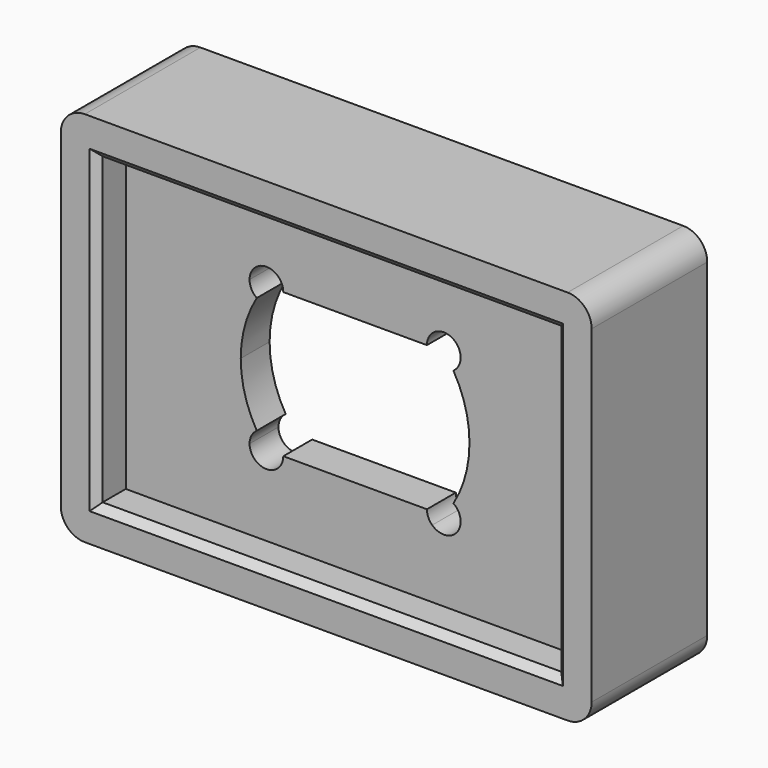
from build123d import *

# Parameters (mm, degrees)
F0_W     = 38.1
F0_H     = 25.3
F1_DEPTH = 3
F0_W_2   = 44.1
F0_H_2   = 31.3
F2_DEPTH = 6
F3_DEPTH = 6
F4_SIZE  = 0.6
F5_R     = 2


# Not quite as in the source:
# - a feature names something its author has since deleted; it is built from what else it names


with BuildPart() as f1:
    # F0 (on Front) → F1 (new body)
    with BuildSketch(Plane.XZ):
        Rectangle(F0_W, F0_H)
        with BuildLine():
            ThreePointArc((-8.6746757864, 9), (0, 12.5), (8.6746757864, 9))
            Line((8.6746757864, 9), (12.5, 9))
            Line((12.5, 9), (12.5, 0))
            Line((12.5, 0), (12.5, -9))
            Line((12.5, -9), (8.6746757864, -9))
            ThreePointArc((8.6746757864, -9), (0, -12.5), (-8.6746757864, -9))
            Line((-8.6746757864, -9), (-12.5, -9))
            Line((-12.5, -9), (-12.5, 0))
            Line((-12.5, 0), (-12.5, 9))
            Line((-12.5, 9), (-8.6746757864, 9))
        make_face(mode=Mode.SUBTRACT)
        with BuildLine():
            ThreePointArc((-3.0413812651, 9), (0, 9.5), (3.0413812651, 9))
            Line((3.0413812651, 9), (8.6746757864, 9))
            ThreePointArc((8.6746757864, 9), (0, 12.5), (-8.6746757864, 9))
            Line((-8.6746757864, 9), (-3.0413812651, 9))
        make_face()
        with BuildLine():
            ThreePointArc((12.5, 0), (11.5039872942, -4.8896090165), (8.6746757864, -9))
            Line((8.6746757864, -9), (12.5, -9))
            Line((12.5, -9), (12.5, 0))
        make_face()
        with BuildLine():
            Line((8.6746757864, -9), (3.0413812651, -9))
            ThreePointArc((3.0413812651, -9), (0, -9.5), (-3.0413812651, -9))
            Line((-3.0413812651, -9), (-8.6746757864, -9))
            ThreePointArc((-8.6746757864, -9), (0, -12.5), (8.6746757864, -9))
        make_face()
        with BuildLine():
            Line((-12.5, -9), (-8.6746757864, -9))
            ThreePointArc((-8.6746757864, -9), (-11.5039872942, -4.8896090165), (-12.5, 0))
            Line((-12.5, 0), (-12.5, -9))
        make_face()
        with BuildLine():
            Line((-3.0413812651, 9), (3.0413812651, 9))
            ThreePointArc((3.0413812651, 9), (0, 9.5), (-3.0413812651, 9))
        make_face()
        with BuildLine():
            ThreePointArc((-3.0413812651, -9), (0, -9.5), (3.0413812651, -9))
            Line((3.0413812651, -9), (-3.0413812651, -9))
        make_face()
        with BuildLine():
            ThreePointArc((-6.4036735124, 7.0173332219), (-4.8254540539, 8.1832141102), (-3.0413812651, 9))
            Line((-3.0413812651, 9), (-8.6746757864, 9))
            ThreePointArc((-8.6746757864, 9), (-11.5039872942, 4.8896090165), (-12.5, 0))
            ThreePointArc((-12.5, 0), (-11.5039872942, -4.8896090165), (-8.6746757864, -9))
            Line((-8.6746757864, -9), (-3.0413812651, -9))
            ThreePointArc((-3.0413812651, -9), (-4.8254540539, -8.1832141102), (-6.4036735124, -7.0173332219))
            ThreePointArc((-6.4036735124, -7.0173332219), (-7.9193096463, -7.2857878881), (-8.7654599313, -6))
            Line((-8.7654599313, -6), (-9.5, -6))
            Line((-9.5, -6), (-9.5, 0))
            Line((-9.5, 0), (-9.5, 6))
            Line((-9.5, 6), (-8.7654599313, 6))
            ThreePointArc((-8.7654599313, 6), (-7.9193096463, 7.2857878881), (-6.4036735124, 7.0173332219))
        make_face()
        with BuildLine():
            Line((9.5, 6), (9.5, 0))
            Line((9.5, 0), (9.5, -6))
            Line((9.5, -6), (8.7654599313, -6))
            ThreePointArc((8.7654599313, -6), (7.9193096463, -7.2857878881), (6.4036735124, -7.0173332219))
            ThreePointArc((6.4036735124, -7.0173332219), (4.8254540539, -8.1832141102), (3.0413812651, -9))
            Line((3.0413812651, -9), (8.6746757864, -9))
            ThreePointArc((8.6746757864, -9), (11.5039872942, -4.8896090165), (12.5, 0))
            ThreePointArc((12.5, 0), (11.5039872942, 4.8896090165), (8.6746757864, 9))
            Line((8.6746757864, 9), (3.0413812651, 9))
            ThreePointArc((3.0413812651, 9), (4.8254540539, 8.1832141102), (6.4036735124, 7.0173332219))
            ThreePointArc((6.4036735124, 7.0173332219), (7.9193096463, 7.2857878881), (8.7654599313, 6))
            Line((8.7654599313, 6), (9.5, 6))
        make_face()
        with BuildLine():
            Line((9.5, -6), (9.5, 0))
            ThreePointArc((9.5, 0), (9.1607649693, -2.5160256709), (8.1672873313, -4.852362069))
            ThreePointArc((8.1672873313, -4.852362069), (8.6069425852, -5.3529135915), (8.7654599313, -6))
            Line((8.7654599313, -6), (9.5, -6))
        make_face()
        with BuildLine():
            ThreePointArc((-8.7654599313, -6), (-8.6069425852, -5.3529135915), (-8.1672873313, -4.852362069))
            ThreePointArc((-8.1672873313, -4.852362069), (-9.1607649693, -2.5160256709), (-9.5, 0))
            Line((-9.5, 0), (-9.5, -6))
            Line((-9.5, -6), (-8.7654599313, -6))
        make_face()
        with BuildLine():
            ThreePointArc((-9.5, 0), (-9.1607649693, 2.5160256709), (-8.1672873313, 4.852362069))
            ThreePointArc((-8.1672873313, 4.852362069), (-8.6069425852, 5.3529135915), (-8.7654599313, 6))
            Line((-8.7654599313, 6), (-9.5, 6))
            Line((-9.5, 6), (-9.5, 0))
        make_face()
        with BuildLine():
            ThreePointArc((8.1672873313, 4.852362069), (9.1607649693, 2.5160256709), (9.5, 0))
            Line((9.5, 0), (9.5, 6))
            Line((9.5, 6), (8.7654599313, 6))
            ThreePointArc((8.7654599313, 6), (8.6069425852, 5.3529135915), (8.1672873313, 4.852362069))
        make_face()
        with BuildLine():
            ThreePointArc((-12.5, 0), (-11.5039872942, 4.8896090165), (-8.6746757864, 9))
            Line((-8.6746757864, 9), (-12.5, 9))
            Line((-12.5, 9), (-12.5, 0))
        make_face()
        with BuildLine():
            Line((12.5, 9), (8.6746757864, 9))
            ThreePointArc((8.6746757864, 9), (11.5039872942, 4.8896090165), (12.5, 0))
            Line((12.5, 0), (12.5, 9))
        make_face()
        with BuildLine():
            ThreePointArc((5.9654599313, 6), (6.0796720432, 6.5538497149), (6.4036735124, 7.0173332219))
            ThreePointArc((6.4036735124, 7.0173332219), (4.8254540539, 8.1832141102), (3.0413812651, 9))
            Line((3.0413812651, 9), (-3.0413812651, 9))
            ThreePointArc((-3.0413812651, 9), (-4.8254540539, 8.1832141102), (-6.4036735124, 7.0173332219))
            ThreePointArc((-6.4036735124, 7.0173332219), (-6.0796720432, 6.5538497149), (-5.9654599313, 6))
            Line((-5.9654599313, 6), (5.9654599313, 6))
        make_face()
        with BuildLine():
            ThreePointArc((3.0413812651, -9), (4.8254540539, -8.1832141102), (6.4036735124, -7.0173332219))
            ThreePointArc((6.4036735124, -7.0173332219), (6.0796720432, -6.5538497149), (5.9654599313, -6))
            Line((5.9654599313, -6), (-5.9654599313, -6))
            ThreePointArc((-5.9654599313, -6), (-6.0796720432, -6.5538497149), (-6.4036735124, -7.0173332219))
            ThreePointArc((-6.4036735124, -7.0173332219), (-4.8254540539, -8.1832141102), (-3.0413812651, -9))
            Line((-3.0413812651, -9), (3.0413812651, -9))
        make_face()
    extrude(amount=F1_DEPTH)

    # F0 (on Front) → F2 (join)
    with BuildSketch(Plane.XZ):
        Rectangle(F0_W_2, F0_H_2)
        Rectangle(F0_W, F0_H, mode=Mode.SUBTRACT)
    extrude(amount=F2_DEPTH)

    # F0 (on Front) → F3 (join)
    with BuildSketch(Plane.XZ):
        Rectangle(F0_W_2, F0_H_2)
        Rectangle(F0_W, F0_H, mode=Mode.SUBTRACT)
    extrude(amount=-F3_DEPTH)

    # F4
    f4_edges = [f1.edges().sort_by_distance(p)[0] for p in [
        (-19.05, -6, 0),
        (0, -6, -12.65),
        (0, -6, 12.65),
        (19.05, -6, 0),
    ]]
    chamfer(f4_edges, length=F4_SIZE)

    # F5
    f5_edges = [f1.edges().sort_by_distance(p)[0] for p in [
        (22.05, 0, 15.65),
        (22.05, 0, -15.65),
        (-22.05, 0, -15.65),
        (-22.05, 0, 15.65),
    ]]
    fillet(f5_edges, radius=F5_R)


solid = f1.part
